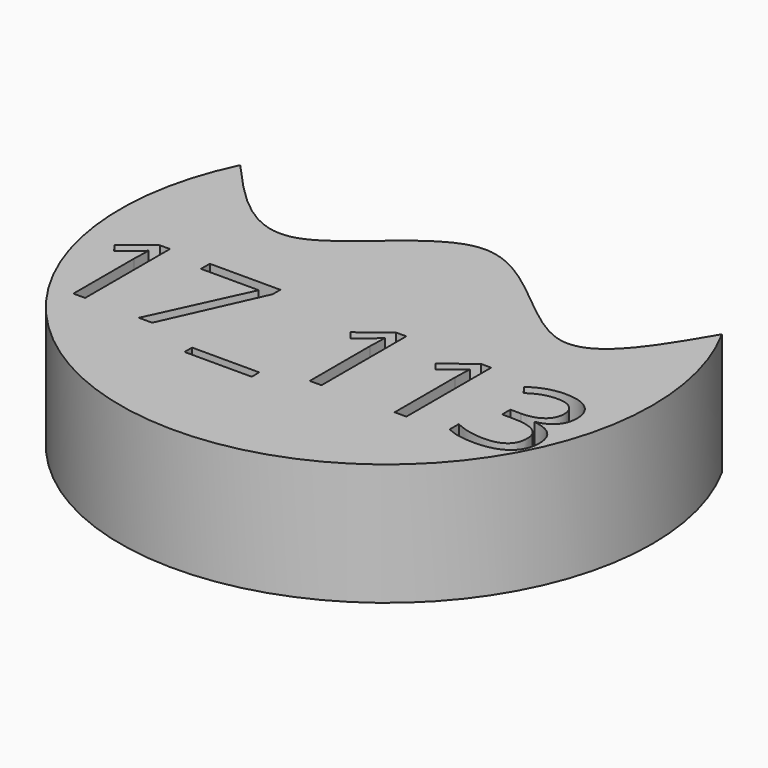
from build123d import *

# Parameters (mm, degrees)
F1_DEPTH     = 25.4
F2_TEXT_SIZE = 22.8950520977
F3_DEPTH     = 25.4
F4_TEXT_SIZE = 30.9507168519
F5_DEPTH     = 25.4


# Not quite as in the source:
# - Text() gives the source's letters only with a copy of the font that has no kerning and outlines rounded to 1/6400 em; it was checked with that copy


with BuildPart() as f1:
    # F0 (on Top) → F1 (new body)
    with BuildSketch(Plane.XY):
        with BuildLine():
            add(Edge.make_bspline(
                [(-49.860174449, 24.2349281431), (-42.5056869401, 16.0244083683), (-27.1130149638, -1.1469472462), (-0.3542706407, 40.9341641024), (30.7250802137, -3.8026309069), (42.9346887301, 17.0002532622), (48.6004362572, 26.6714516628)],
                knots=[0, 0, 0, 0, 0.2374510716, 0.496000038, 0.7654112853, 1, 1, 1, 1], degree=3))
            ThreePointArc((-49.860174449, 24.2349281431), (1.371457908, -55.4210054167), (48.6004362572, 26.6714516628))
        make_face()
    extrude(amount=F1_DEPTH)

    # F2 (on Top) → F3 (join)
    with BuildSketch(Plane.XY):
        with Locations((-37.9270847407, -36.3268144429)):
            Text('17_113', F2_TEXT_SIZE, font='Open Sans', text_align=(TextAlign.LEFT, TextAlign.BOTTOM))
    extrude(amount=F3_DEPTH)

    # F4 (on Top) → F5 (cut)
    with BuildSketch(Plane.XY):
        with Locations((-51.1322796228, -28.0846003443)):
            Text('17_113', F4_TEXT_SIZE, font='Open Sans', text_align=(TextAlign.LEFT, TextAlign.BOTTOM))
    extrude(amount=F5_DEPTH, mode=Mode.SUBTRACT)


solid = f1.part
